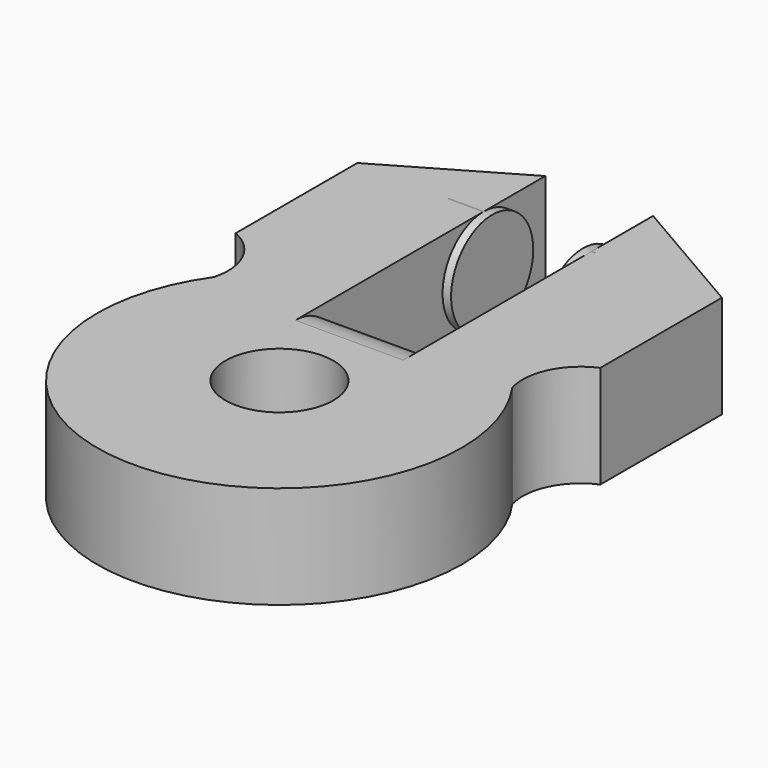
from build123d import *

# Parameters (mm, degrees)
F0_R     = 3.15
F1_DEPTH = 6
F3_START = 22.4
F2_R     = 3
F3_DEPTH = 8.6
F5_START = -52.7
F5_DEPTH = 11
F6_R     = 3
F7_R     = 2.99999


# Not quite as in the source:
# - a fillet or chamfer is up to 0.001 mm smaller than in the source, because OpenCascade refuses the exact size


with BuildPart() as f1:
    # F0 (on Top) → F1 (new body)
    with BuildSketch(Plane.XY):
        with BuildLine():
            Line((24.4793512434, 46.0903614521), (24.4793512434, 48.1638564268))
            ThreePointArc((24.4793512434, 48.1638564268), (21.3598687714, 46.599431642), (18.9135639574, 44.1106189618))
            ThreePointArc((18.9135639574, 44.1106189618), (27.6293512434, 27.3403614521), (36.3451385294, 44.1106189618))
            ThreePointArc((36.3451385294, 44.1106189618), (33.8988337153, 46.599431642), (30.7793512434, 48.1638564268))
            Line((30.7793512434, 48.1638564268), (30.7793512434, 46.0903614521))
            Line((30.7793512434, 46.0903614521), (27.6293512434, 46.0903614521))
            Line((27.6293512434, 46.0903614521), (24.4793512434, 46.0903614521))
        make_face()
        with Locations((27.6293512434, 37.9903614521)):
            Circle(F0_R, mode=Mode.SUBTRACT)
        with BuildLine():
            ThreePointArc((18.9135639574, 44.1106189618), (21.3598687714, 46.599431642), (24.4793512434, 48.1638564268))
            Line((24.4793512434, 48.1638564268), (24.4793512434, 61.3403614521))
            Line((24.4793512434, 61.3403614521), (16.9793512434, 56.9903614521))
            Line((16.9793512434, 56.9903614521), (16.9793512434, 48.1108582074))
            ThreePointArc((16.9793512434, 48.1108582074), (18.6903086712, 46.4704086219), (18.9135639574, 44.1106189618))
        make_face()
        with BuildLine():
            ThreePointArc((30.7793512434, 48.1638564268), (33.8988337153, 46.599431642), (36.3451385294, 44.1106189618))
            ThreePointArc((36.3451385294, 44.1106189618), (36.5683938155, 46.4704086219), (38.2793512434, 48.1108582074))
            Line((38.2793512434, 48.1108582074), (38.2793512434, 56.9903614521))
            Line((38.2793512434, 56.9903614521), (30.7793512434, 61.3403614521))
            Line((30.7793512434, 61.3403614521), (30.7793512434, 48.1638564268))
        make_face()
    extrude(amount=F1_DEPTH)

    # F2 (on Right) → F3 (join)
    with BuildSketch(Plane.YZ.offset(F3_START)):
        with Locations((56.8403841853, 3.0001187697)):
            Circle(F2_R)
    extrude(amount=F3_DEPTH)

    # F4 (on Front) → F5 (cut)
    with BuildSketch(Plane.XZ.offset(F5_START)):
        Polygon((30.2794827968, -0.6592939026), (30.2794827968, 3.0006368179), (30.2794827968, 6.7412233911), (24.9780313224, 6.7412233911), (24.9780313224, -0.6592939026), align=None)
    extrude(amount=-F5_DEPTH, mode=Mode.SUBTRACT)

    # F6
    f6_edges = [f1.edges().sort_by_distance(p)[0] for p in [
        (27.629351, 46.090361, 6),
    ]]
    fillet(f6_edges, radius=F6_R)

    # F7 (radius 3 in the source; OpenCascade refuses exactly that, so slightly less here)
    f7_edges = [f1.edges().sort_by_distance(p)[0] for p in [
        (27.629351, 46.090361, 0),
    ]]
    fillet(f7_edges, radius=F7_R)


solid = f1.part
